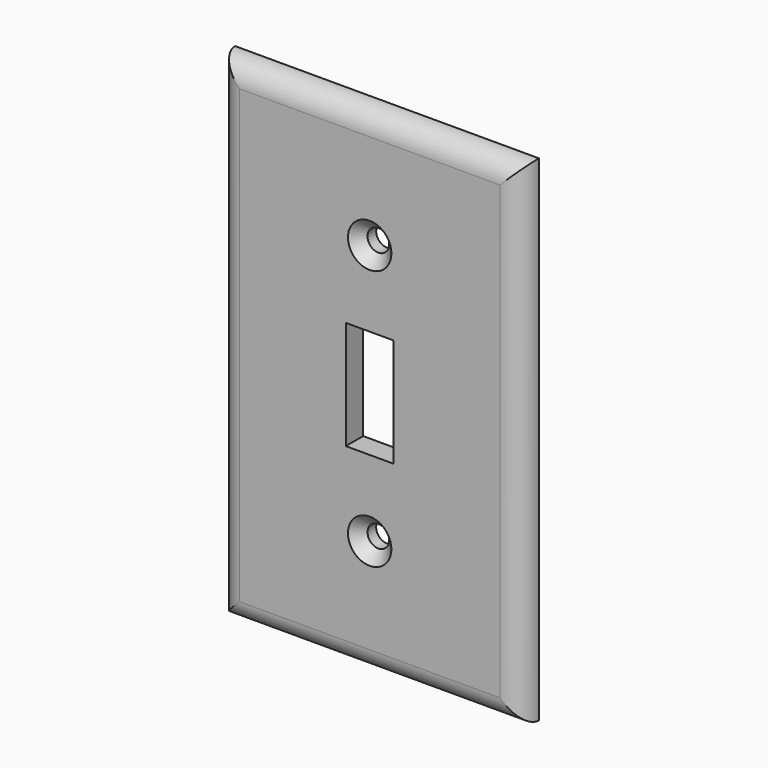
from build123d import *

# Parameters (mm, degrees)
F0_W           = 70
F0_H           = 114
F0_R           = 2.5
F0_W_2         = 11
F0_H_2         = 25
F1_DEPTH       = 5
F2_T           = -2.5
F4_D           = 5
F4_CSINK_D     = 10
F4_CSINK_ANGLE = 90
F5_R           = 4.99999


# Not quite as in the source:
# - a fillet or chamfer is up to 0.001 mm smaller than in the source, because OpenCascade refuses the exact size


with BuildPart() as f1:
    # F0 (on Front) → F1 (new body)
    with BuildSketch(Plane.XZ):
        Rectangle(F0_W, F0_H)
        with Locations((0, -30)):
            Circle(F0_R, mode=Mode.SUBTRACT)
        Rectangle(F0_W_2, F0_H_2, mode=Mode.SUBTRACT)
        with Locations((0, 30)):
            Circle(F0_R, mode=Mode.SUBTRACT)
    extrude(amount=F1_DEPTH)

    # F2
    f2_openings = [f1.faces().sort_by_distance(p)[0] for p in [
        (0, 0, -55.662241),
    ]]
    offset(amount=F2_T, openings=f2_openings, kind=Kind.INTERSECTION)

    # F4 (through all)
    with Locations(Plane.XZ.offset(5)):
        with Locations((0, 30), (0, -30)):
            CounterSinkHole(F4_D / 2, F4_CSINK_D / 2, counter_sink_angle=F4_CSINK_ANGLE)

    # F5 (radius 5 in the source; OpenCascade refuses exactly that, so slightly less here)
    f5_edges = [f1.edges().sort_by_distance(p)[0] for p in [
        (-35, -5, 0),
        (0, -5, 57),
        (35, -5, 0),
        (0, -5, -57),
    ]]
    fillet(f5_edges, radius=F5_R)


solid = f1.part
